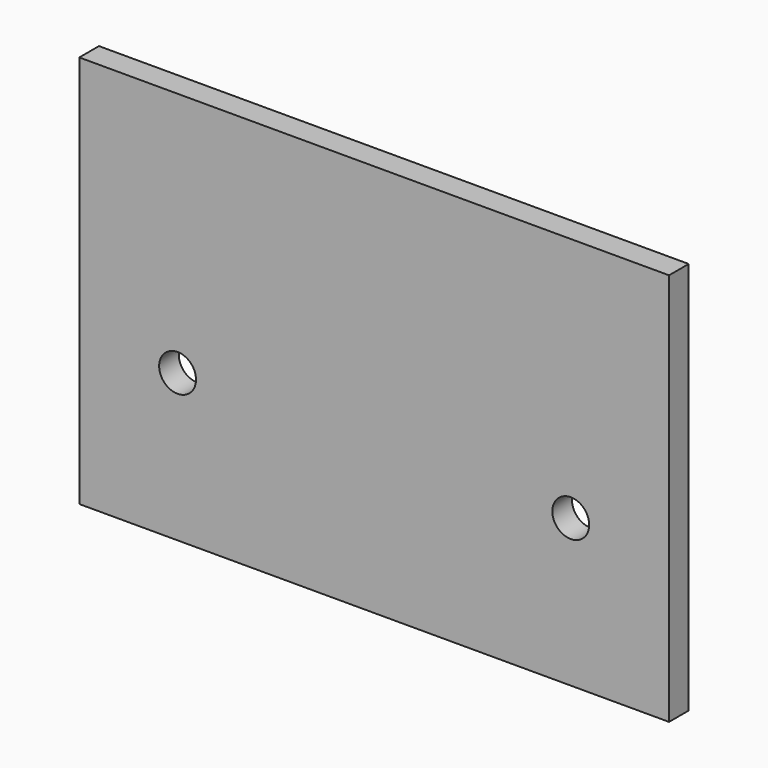
from build123d import *

# Parameters (mm, degrees)
F0_W     = 76.2
F0_H     = 50.8
F1_DEPTH = 1.5875
F2_R     = 2.38125
F4_DEPTH = 3.175
F3_R     = 2.38125
F5_DEPTH = 3.175


# Not quite as in the source:
# - a length typed as a fraction of an inch, garbled in the dataset ("3 / 203.2 mm" for 3/8 in), is restored


with BuildPart() as f1:
    # F0 (on Front) → F1 (new body, symmetric)
    with BuildSketch(Plane.XZ):
        Rectangle(F0_W, F0_H)
    extrude(amount=F1_DEPTH, both=True)

    # F2 (on face) → F4 (cut, through all)
    with BuildSketch(Plane.XZ.offset(1.5875)):
        with Locations((-25.4, -6.35)):
            Circle(F2_R)
    extrude(amount=-F4_DEPTH, mode=Mode.SUBTRACT)

    # F3 (on face) → F5 (cut, through all)
    with BuildSketch(Plane.XZ.offset(1.5875)):
        with Locations((25.4, -6.35)):
            Circle(F3_R)
    extrude(amount=-F5_DEPTH, mode=Mode.SUBTRACT)


solid = f1.part
